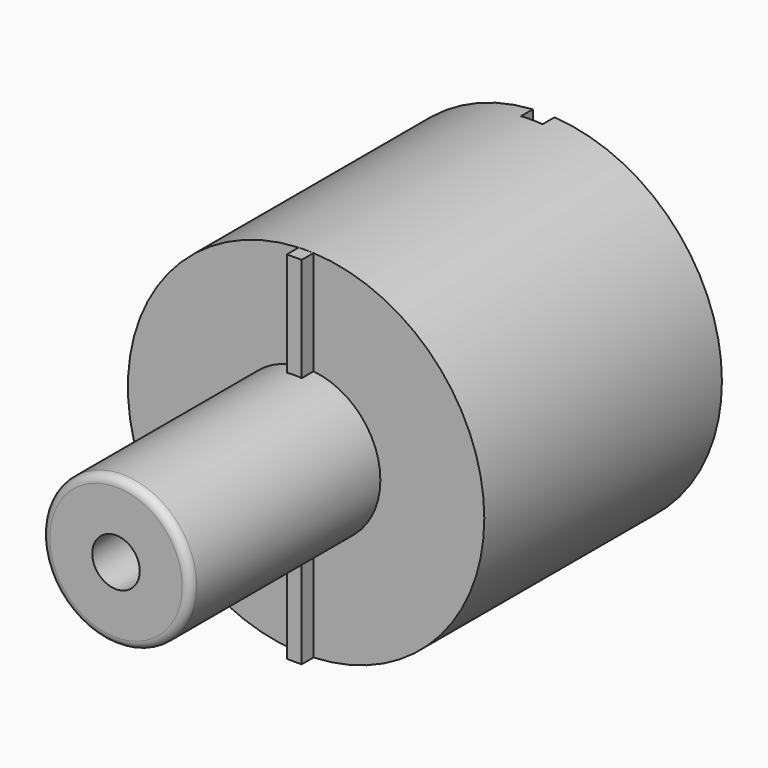
from build123d import *

# Parameters (mm, degrees)
F0_R      = 19.05
F1_DEPTH  = 31.75
F2_R      = 7.9375
F3_DEPTH  = 25.4
F4_R      = 0.8584943428
F6_DEPTH  = 1.5875
F8_DEPTH  = 1.5875
F11_R     = 7.9375
F12_DEPTH = 25.4
F9_R      = 2.54
F13_DEPTH = 31.75
F14_DEPTH = 1.5875


with BuildPart() as f1:
    # F0 (on Front) → F1 (new body)
    with BuildSketch(Plane.XZ):
        Circle(F0_R)
    extrude(amount=F1_DEPTH)

    # F2 (on face) → F3 (join)
    with BuildSketch(Plane.XZ.offset(31.75)):
        Circle(F2_R)
    extrude(amount=F3_DEPTH)

    # F4
    f4_edges = [f1.edges().sort_by_distance(p)[0] for p in [
        (-7.9375, -57.15, 0),
    ]]
    fillet(f4_edges, radius=F4_R)

    # F5 (on face) → F6 (join)
    with BuildSketch(Plane.XZ.offset(31.75)):
        with BuildLine():
            Line((0.79375, 19.0334563581), (-0.79375, 19.0334563581))
            Line((-0.79375, 19.0334563581), (-0.79375, 7.897712782))
            ThreePointArc((-0.79375, 7.897712782), (0, 7.9375), (0.79375, 7.897712782))
            Line((0.79375, 7.897712782), (0.79375, 19.0334563581))
        make_face()
    extrude(amount=F6_DEPTH)

    # F7 (on face) → F8 (join)
    with BuildSketch(Plane.XZ.offset(31.75)):
        with BuildLine():
            Line((-0.79375, -7.897712782), (-0.79375, -19.0334563581))
            Line((-0.79375, -19.0334563581), (0.79375, -19.0334563581))
            Line((0.79375, -19.0334563581), (0.79375, -7.897712782))
            ThreePointArc((0.79375, -7.897712782), (0, -7.9375), (-0.79375, -7.897712782))
        make_face()
    extrude(amount=F8_DEPTH)

    # F11 (on face) → F12 (cut)
    with BuildSketch(Plane(origin=(0, 0, 0), x_dir=(-1, 0, 0), z_dir=(0, 1, 0))):
        Circle(F11_R)
    extrude(amount=-F12_DEPTH, mode=Mode.SUBTRACT)

    # F9 (on face) → F13 (cut)
    with BuildSketch(Plane.XZ.offset(57.15)):
        Circle(F9_R)
    extrude(amount=-F13_DEPTH, mode=Mode.SUBTRACT)

    # F10 (on face) → F14 (cut)
    with BuildSketch(Plane(origin=(0, 0, 0), x_dir=(-1, 0, 0), z_dir=(0, 1, 0))):
        with BuildLine():
            ThreePointArc((1.1575095176, 19.0148013851), (0, 19.05), (-1.1575095176, 19.0148013851))
            Line((-1.1575095176, 19.0148013851), (-1.1575095176, -19.0148013851))
            ThreePointArc((-1.1575095176, -19.0148013851), (0, -19.05), (1.1575095176, -19.0148013851))
            Line((1.1575095176, -19.0148013851), (1.1575095176, 19.0148013851))
        make_face()
    extrude(amount=-F14_DEPTH, mode=Mode.SUBTRACT)


solid = f1.part
